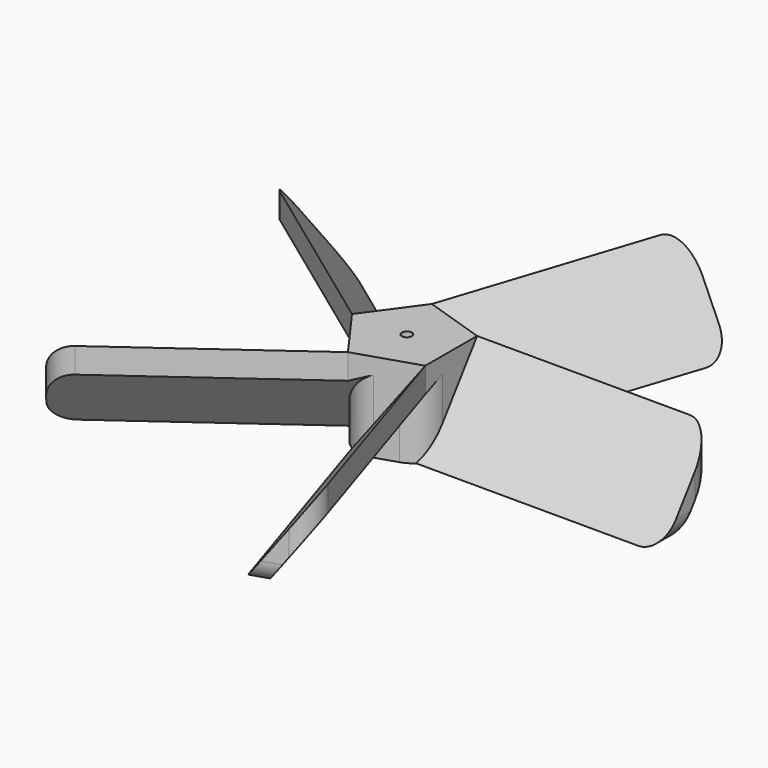
from build123d import *

# Parameters (mm, degrees)
F0_R          = 1.0795
F1_DEPTH      = 19.05
F3_DEPTH      = 50.8
F5_DEPTH      = 50.8
F7_DEPTH      = 50.8
F9_DEPTH      = 50.8
F11_DEPTH     = 50.8
F12_R         = 6.35
F13_T1_DEPTH  = 30.801632633
F13_T3_DEPTH  = 29.3245158286
F13_T5_DEPTH  = 29.3245158286
F13_T7_DEPTH  = 29.3245158286
F13_T9_DEPTH  = 29.3245158286
F13_T11_DEPTH = 29.3245158286


# Not quite as in the source:
# - a fillet or chamfer that OpenCascade refuses, or shapes differently, is made with other operations: its cross-section is extruded or revolved along the edge and cut away or added


with BuildPart() as f1:
    # F0 (on Top) → F1 (new body)
    with BuildSketch(Plane.XY):
        Polygon((-3.666268911, -11.1881585915), (9.5076317344, -6.9441600789), (9.5423084754, 6.8964316395), (-3.6101607654, 11.2063892332), (-11.7735105333, 0.0294977978), align=None)
        Circle(F0_R, mode=Mode.SUBTRACT)
    extrude(amount=F1_DEPTH)

    # F2 (on face) → F3 (join)
    with BuildSketch(Plane(origin=(-7.7198897222, -5.5793303969, 0), x_dir=(0.5857564721, -0.8104871099, 0), z_dir=(-0.8104871099, -0.5857564721, 0))):
        Polygon((6.9203175793, 19.05), (-6.9203175793, 0), (-2.9958017507, 0), (6.9203175793, 13.648367367), align=None)
    extrude(amount=F3_DEPTH)

    # F4 (on face) → F5 (join)
    with BuildSketch(Plane(origin=(2.9206814117, -9.0661593352, 0), x_dir=(0.9518277517, 0.3066332191, 0), z_dir=(0.3066332191, -0.9518277517, 0))):
        Polygon((6.9203175793, 19.05), (-6.9203175793, 0), (-2.9958017507, 0), (6.9203175793, 13.648367367), align=None)
    extrude(amount=F5_DEPTH)

    # F6 (on face) → F7 (join)
    with BuildSketch(Plane(origin=(9.5249701049, -0.0238642197, 0), x_dir=(0.0025054299, 0.9999968614, 0), z_dir=(0.9999968614, -0.0025054299, 0))):
        Polygon((6.9203175793, 19.05), (-6.9203175793, 0), (-2.9958017507, 0), (6.9203175793, 13.648367367), align=None)
    extrude(amount=F7_DEPTH)

    # F8 (on face) → F9 (join)
    with BuildSketch(Plane(origin=(2.966073855, 9.0514104363, 0), x_dir=(-0.9502793109, 0.3113988299, 0), z_dir=(0.3113988299, 0.9502793109, 0))):
        Polygon((6.9203175793, 19.05), (-6.9203175793, 0), (-2.9958017507, 0), (6.9203175793, 13.648367367), align=None)
    extrude(amount=F9_DEPTH)

    # F10 (on face) → F11 (join)
    with BuildSketch(Plane(origin=(-7.6918356494, 5.6179435155, 0), x_dir=(-0.5898103428, -0.8075418005, 0), z_dir=(-0.8075418005, 0.5898103428, 0))):
        Polygon((6.9203175793, 19.05), (-6.9203175793, 0), (-2.9958017507, 0), (6.9203175793, 13.648367367), align=None)
    extrude(amount=F11_DEPTH)

    # F12
    f12_edges = [f1.edges().sort_by_distance(p)[0] for p in [
        (-3.610161, 11.206389, 6.824184),
        (-11.773511, 0.029498, 6.824184),
        (-3.666269, -11.188159, 6.824184),
        (9.507632, -6.94416, 6.824184),
        (9.542308, 6.896432, 6.824184),
    ]]
    fillet(f12_edges, radius=F12_R)

    # F13: fillet of radius 5.08 on 10 edges, made by hand

    # F13_s2 → F13_t1 (cut)
    with BuildSketch(Plane.XY.offset(0.948367367)):
        with BuildLine():
            ThreePointArc((-49.800397455, 34.09417556), (-50.7175171639, 30.3158253164), (-48.6943216503, 26.9956266721))
            Line((-48.6943216503, 26.9956266721), (-52.7966339966, 29.9918632137))
            Line((-52.7966339966, 29.9918632137), (-49.800397455, 34.09417556))
        make_face()
        with BuildLine():
            ThreePointArc((-47.8146569743, -36.8273128564), (-44.5046379302, -38.8671199678), (-40.7217395774, -37.9689444966))
            Line((-40.7217395774, -37.9689444966), (-44.8390140959, -40.9445873749))
            Line((-44.8390140959, -40.9445873749), (-47.8146569743, -36.8273128564))
        make_face()
        with BuildLine():
            ThreePointArc((20.2493142845, -56.8547066196), (23.2121382661, -54.3370265013), (23.5269025104, -50.4617248879))
            Line((23.5269025104, -50.4617248879), (25.0845992633, -55.2970098667))
            Line((25.0845992633, -55.2970098667), (20.2493142845, -56.8547066196))
        make_face()
        with BuildLine():
            ThreePointArc((60.329421451, 1.6891717451), (58.8505283301, 5.2849907424), (55.2621649789, 6.7818833849))
            Line((55.2621649789, 6.7818833849), (60.3421490348, 6.769155801))
            Line((60.3421490348, 6.769155801), (60.329421451, 1.6891717451))
        make_face()
        with BuildLine():
            ThreePointArc((10.6269937385, 54.6531593275), (13.1594884979, 57.6033304103), (17.0363186938, 57.8986721709))
            Line((17.0363186938, 57.8986721709), (12.2088997945, 59.4805782269))
            Line((12.2088997945, 59.4805782269), (10.6269937385, 54.6531593275))
        make_face()
    extrude(amount=F13_T1_DEPTH, mode=Mode.SUBTRACT)

    # F13_s4 → F13_t3 (cut)
    with BuildSketch(Plane(origin=(11.5722662379, 15.8442265835, 0), x_dir=(0, 0, 1), z_dir=(-0.5898103428, -0.8075418005, 0))):
        with BuildLine():
            ThreePointArc((0, 55.245), (1.4878975516, 58.8371024484), (5.08, 60.325))
            Line((5.08, 60.325), (0, 60.325))
            Line((0, 60.325), (0, 55.245))
        make_face()
    extrude(amount=F13_T3_DEPTH, mode=Mode.SUBTRACT)

    # F13_s6 → F13_t5 (cut)
    with BuildSketch(Plane(origin=(-11.492728007, 15.9020144909, 0), x_dir=(0, 0, 1), z_dir=(0.5857564721, -0.8104871099, 0))):
        with BuildLine():
            ThreePointArc((0, 55.245), (1.4878975516, 58.8371024484), (5.08, 60.325))
            Line((5.08, 60.325), (0, 60.325))
            Line((0, 60.325), (0, 55.245))
        make_face()
    extrude(amount=F13_T5_DEPTH, mode=Mode.SUBTRACT)

    # F13_s8 → F13_t7 (cut)
    with BuildSketch(Plane(origin=(-18.6751627697, -6.0162411386, 0), x_dir=(0, 0, 1), z_dir=(0.9518277517, 0.3066332191, 0))):
        with BuildLine():
            ThreePointArc((0, 55.245), (1.4878975516, 58.8371024484), (5.08, 60.325))
            Line((5.08, 60.325), (0, 60.325))
            Line((0, 60.325), (0, 55.245))
        make_face()
    extrude(amount=F13_T7_DEPTH, mode=Mode.SUBTRACT)

    # F13_s10 → F13_t9 (cut)
    with BuildSketch(Plane(origin=(-0.0491573301, -19.620255999, 0), x_dir=(0, 0, 1), z_dir=(0.0025054299, 0.9999968614, 0))):
        with BuildLine():
            ThreePointArc((0, 55.245), (1.4878975516, 58.8371024484), (5.08, 60.325))
            Line((5.08, 60.325), (0, 60.325))
            Line((0, 60.325), (0, 55.245))
        make_face()
    extrude(amount=F13_T9_DEPTH, mode=Mode.SUBTRACT)

    # F13_s12 → F13_t11 (cut)
    with BuildSketch(Plane(origin=(18.6447818689, -6.1097439368, 0), x_dir=(0, 0, 1), z_dir=(-0.9502793109, 0.3113988299, 0))):
        with BuildLine():
            ThreePointArc((0, 55.245), (1.4878975516, 58.8371024484), (5.08, 60.325))
            Line((5.08, 60.325), (0, 60.325))
            Line((0, 60.325), (0, 55.245))
        make_face()
    extrude(amount=F13_T11_DEPTH, mode=Mode.SUBTRACT)


solid = f1.part
